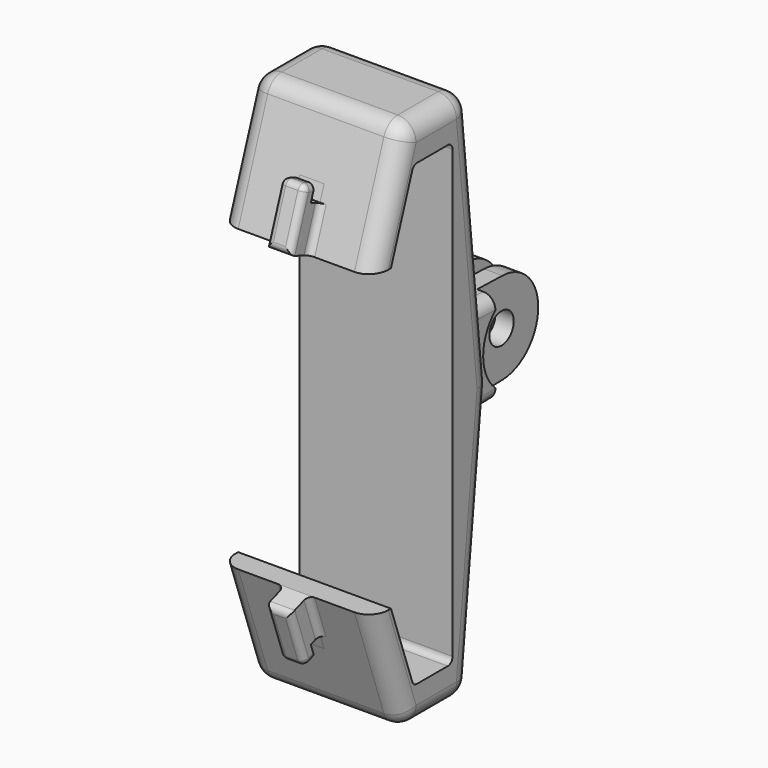
from build123d import *

# Parameters (mm, degrees)
F1_DEPTH      = 12.5
F3_DEPTH      = 7.5
F2_R          = 2.5
F4_DEPTH      = 4.5
F5_DEPTH      = 1.5
F6_R          = 3
F7_R          = 1.99999
F8_W          = 4
F8_H          = 7
F8_H_2        = 2.5
F9_DEPTH      = 4
F10_DEPTH     = 2
F11_T1_DEPTH  = 7
F11_T3_DEPTH  = 7
F11_T5_DEPTH  = 25
F11_T7_DEPTH  = 7
F11_T9_DEPTH  = 7
F11_T11_DEPTH = 9
F11_T13_DEPTH = 11
F11_T15_DEPTH = 2
F11_T17_DEPTH = 11
F11_T19_DEPTH = 11
F11_T21_DEPTH = 11
F11_T26_DEPTH = 1.02
F11_S31_W     = 1.02
F11_S31_H     = 1.02
F11_T32_DEPTH = 1.02
F11_T38_DEPTH = 1.02
F11_S43_W     = 1.02
F11_S43_H     = 1.02
F11_T44_DEPTH = 1.02
F11_T50_DEPTH = 3.5
F11_T55_DEPTH = 3.5
F11_T60_DEPTH = 3.5
F11_T65_DEPTH = 3.5


# Not quite as in the source:
# - a fillet or chamfer that OpenCascade refuses, or shapes differently, is made with other operations: its cross-section is extruded or revolved along the edge and cut away or added
# - two fillets or chamfers of one size are made in one step
# - a fillet or chamfer is up to 0.001 mm smaller than in the source, because OpenCascade refuses the exact size
# - a pattern or mirror of a feature is missing from the dataset's text; its kind, count and spacing are read off the source's solid


with BuildPart() as f1:
    # F0 (on Right) → F1 (new body, symmetric)
    with BuildSketch(Plane.YZ):
        Polygon((-8, 37.5), (0, 37.5), (0, -37.5), (-8, -37.5), (-12.6, -24.5), (-16.312652284, -24.5), (-9.589575361, -43.5), (3.5, -43.5), (8, 0), (3.5, 43.5), (-9.589575361, 43.5), (-16.312652284, 24.5), (-12.6, 24.5), align=None)
    extrude(amount=F1_DEPTH, both=True)

    # F2 (on Right) → F3 (join, symmetric)
    with BuildSketch(Plane.YZ):
        with BuildLine():
            ThreePointArc((15, -5.5901699437), (12.5, 0), (15, 5.5901699437))
            Line((15, 5.5901699437), (15, 7.6335005515))
            Line((15, 7.6335005515), (7.189168859, 7.8380343632))
            Line((7.189168859, 7.8380343632), (8, 0))
            Line((8, 0), (7.189168859, -7.8380343632))
            Line((7.189168859, -7.8380343632), (15, -7.6335005515))
            Line((15, -7.6335005515), (15, -5.5901699437))
        make_face()
    extrude(amount=F3_DEPTH, both=True)

    # F2 (on Right) → F4 (join, symmetric)
    with BuildSketch(Plane.YZ):
        with BuildLine():
            ThreePointArc((15, 5.5901699437), (17.4157731381, 7.0407223725), (20.1963271123, 7.4974299373))
            Line((20.1963271123, 7.4974299373), (15, 7.6335005515))
            Line((15, 7.6335005515), (15, 5.5901699437))
        make_face()
        with BuildLine():
            ThreePointArc((20.1963271123, -7.4974299373), (25.3722645757, -5.2334284488), (27.5, 0))
            ThreePointArc((27.5, 0), (25.3722645757, 5.2334284488), (20.1963271123, 7.4974299373))
            ThreePointArc((20.1963271123, 7.4974299373), (17.4157731381, 7.0407223725), (15, 5.5901699437))
            Line((15, 5.5901699437), (15, -5.5901699437))
            ThreePointArc((15, -5.5901699437), (17.4157731381, -7.0407223725), (20.1963271123, -7.4974299373))
        make_face()
        with Locations((20, 0)):
            Circle(F2_R, mode=Mode.SUBTRACT)
        with BuildLine():
            Line((15, -5.5901699437), (15, 5.5901699437))
            ThreePointArc((15, 5.5901699437), (12.5, 0), (15, -5.5901699437))
        make_face()
        with BuildLine():
            Line((15, -7.6335005515), (20.1963271123, -7.4974299373))
            ThreePointArc((20.1963271123, -7.4974299373), (17.4157731381, -7.0407223725), (15, -5.5901699437))
            Line((15, -5.5901699437), (15, -7.6335005515))
        make_face()
    extrude(amount=F4_DEPTH, both=True)

    # F2 (on Right) → F5 (cut, symmetric)
    with BuildSketch(Plane.YZ):
        with BuildLine():
            ThreePointArc((15, 5.5901699437), (17.4157731381, 7.0407223725), (20.1963271123, 7.4974299373))
            Line((20.1963271123, 7.4974299373), (15, 7.6335005515))
            Line((15, 7.6335005515), (15, 5.5901699437))
        make_face()
        with BuildLine():
            Line((15, -7.6335005515), (20.1963271123, -7.4974299373))
            ThreePointArc((20.1963271123, -7.4974299373), (17.4157731381, -7.0407223725), (15, -5.5901699437))
            Line((15, -5.5901699437), (15, -7.6335005515))
        make_face()
        with BuildLine():
            ThreePointArc((20.1963271123, -7.4974299373), (25.3722645757, -5.2334284488), (27.5, 0))
            ThreePointArc((27.5, 0), (25.3722645757, 5.2334284488), (20.1963271123, 7.4974299373))
            ThreePointArc((20.1963271123, 7.4974299373), (17.4157731381, 7.0407223725), (15, 5.5901699437))
            Line((15, 5.5901699437), (15, -5.5901699437))
            ThreePointArc((15, -5.5901699437), (17.4157731381, -7.0407223725), (20.1963271123, -7.4974299373))
        make_face()
        with Locations((20, 0)):
            Circle(F2_R, mode=Mode.SUBTRACT)
        with BuildLine():
            Line((15, -5.5901699437), (15, 5.5901699437))
            ThreePointArc((15, 5.5901699437), (12.5, 0), (15, -5.5901699437))
        make_face()
    extrude(amount=F5_DEPTH, both=True, mode=Mode.SUBTRACT)

    # F6
    f6_edges = [f1.edges().sort_by_distance(p)[0] for p in [
        (12.5, 5.75, 21.75),
        (12.5, 5.75, -21.75),
        (12.5, -3.044788, -43.5),
        (12.5, -12.951114, -34),
        (0, -9.589575, -43.5),
        (-12.5, -12.951114, -34),
        (-12.5, 5.75, -21.75),
        (-12.5, -3.044788, -43.5),
        (-12.5, 5.75, 21.75),
        (0, 3.5, 43.5),
        (0, 3.5, -43.5),
        (0, -9.589575, 43.5),
        (-12.5, -3.044788, 43.5),
        (-12.5, -12.951114, 34),
        (12.5, -12.951114, 34),
        (12.5, -3.044788, 43.5),
    ]]
    fillet(f6_edges, radius=F6_R)

    # F7 (radius 2 in the source; OpenCascade refuses exactly that, so slightly less here)
    f7_edges = [f1.edges().sort_by_distance(p)[0] for p in [
        (0, 7.189169, 7.838034),
        (-7.5, 7.594584, 3.919017),
        (-7.5, 7.594584, -3.919017),
        (0, 7.189169, -7.838034),
        (7.5, 7.594584, -3.919017),
        (7.5, 7.594584, 3.919017),
        (7.5, 11.094584, 7.735767),
        (7.5, 11.094584, -7.735767),
        (-7.5, 11.094584, -7.735767),
        (-7.5, 11.094584, 7.735767),
    ]]
    fillet(f7_edges, radius=F7_R)

    # F8 (on face) → F9 (join)
    with BuildSketch(Plane(origin=(0, -22.2020311107, -7.8561033161), x_dir=(1, 0, 0), z_dir=(0, -0.942722273, -0.3335786504))):
        with Locations((0, -21.155143154)):
            Rectangle(F8_W, F8_H)
        with Locations((0, -25.905143154)):
            Rectangle(F8_W, F8_H_2)
    f9 = extrude(amount=F9_DEPTH)

    # F9_copies: F9 across plane
    add(f9.mirror(Plane.XY))

    # F8 (on face) → F10 (cut)
    with BuildSketch(Plane(origin=(0, -22.2020311107, -7.8561033161), x_dir=(1, 0, 0), z_dir=(0, -0.942722273, -0.3335786504))):
        with Locations((0, -25.905143154)):
            Rectangle(F8_W, F8_H_2)
    f10 = extrude(amount=F10_DEPTH, mode=Mode.SUBTRACT)

    # F10_copies: F10 across plane
    add(f10.mirror(Plane.XY), mode=Mode.SUBTRACT)

    # F11: fillet of radius 1 on 20 edges, made by hand

    # F11_s2 → F11_t1 (join)
    with BuildSketch(Plane(origin=(0, 5.8893788266, -16.6438966839), x_dir=(1, 0, 0), z_dir=(0, 0.3335786504, -0.942722273))):
        with BuildLine():
            ThreePointArc((-3, 23.5509775753), (-2.2928932188, 23.8438707941), (-2, 24.5509775753))
            Line((-2, 24.5509775753), (-2, 23.5509775753))
            Line((-2, 23.5509775753), (-3, 23.5509775753))
        make_face()
    extrude(amount=F11_T1_DEPTH)

    # F11_s4 → F11_t3 (join)
    with BuildSketch(Plane(origin=(0, 8.2244293797, -23.2429525948), x_dir=(1, 0, 0), z_dir=(0, -0.3335786504, 0.942722273))):
        with BuildLine():
            ThreePointArc((3, -23.5509775753), (2.2928932188, -23.8438707941), (2, -24.5509775753))
            Line((2, -24.5509775753), (2, -23.5509775753))
            Line((2, -23.5509775753), (3, -23.5509775753))
        make_face()
    extrude(amount=F11_T3_DEPTH)

    # F11_s6 → F11_t5 (join)
    with BuildSketch(Plane.YZ.offset(-12.5)):
        with BuildLine():
            ThreePointArc((-8.2358106314, 36.8335786504), (-7.8703323924, 37.3165716902), (-7.2930883584, 37.5))
            Line((-7.2930883584, 37.5), (-8, 37.5))
            Line((-8, 37.5), (-8.2358106314, 36.8335786504))
        make_face()
        with BuildLine():
            ThreePointArc((-1, 37.5), (-0.2928932188, 37.2071067812), (0, 36.5))
            Line((0, 36.5), (0, 37.5))
            Line((0, 37.5), (-1, 37.5))
        make_face()
        with BuildLine():
            ThreePointArc((0, -36.5), (-0.2928932188, -37.2071067812), (-1, -37.5))
            Line((-1, -37.5), (0, -37.5))
            Line((0, -37.5), (0, -36.5))
        make_face()
        with BuildLine():
            ThreePointArc((-7.2930883584, -37.5), (-7.8703323924, -37.3165716902), (-8.2358106314, -36.8335786504))
            Line((-8.2358106314, -36.8335786504), (-8, -37.5))
            Line((-8, -37.5), (-7.2930883584, -37.5))
        make_face()
    extrude(amount=F11_T5_DEPTH)

    # F11_s8 → F11_t7 (join)
    with BuildSketch(Plane(origin=(0, 5.8893788266, 16.6438966839), x_dir=(1, 0, 0), z_dir=(0, 0.3335786504, 0.942722273))):
        with BuildLine():
            ThreePointArc((-3, -23.5509775753), (-2.2928932188, -23.8438707941), (-2, -24.5509775753))
            Line((-2, -24.5509775753), (-2, -23.5509775753))
            Line((-2, -23.5509775753), (-3, -23.5509775753))
        make_face()
    extrude(amount=F11_T7_DEPTH)

    # F11_s10 → F11_t9 (join)
    with BuildSketch(Plane(origin=(0, 8.2244293797, 23.2429525948), x_dir=(1, 0, 0), z_dir=(0, -0.3335786504, -0.942722273))):
        with BuildLine():
            ThreePointArc((3, 23.5509775753), (2.2928932188, 23.8438707941), (2, 24.5509775753))
            Line((2, 24.5509775753), (2, 23.5509775753))
            Line((2, 23.5509775753), (3, 23.5509775753))
        make_face()
    extrude(amount=F11_T9_DEPTH)

    # F11_s12 → F11_t11 (cut)
    with BuildSketch(Plane.YZ.offset(-4.5)):
        with BuildLine():
            ThreePointArc((-19.140819103, -25.5007359513), (-19.7097214903, -26.0127286381), (-19.7499627255, -26.7770368747))
            Line((-19.7499627255, -26.7770368747), (-20.083541376, -25.8343146018))
            Line((-20.083541376, -25.8343146018), (-19.140819103, -25.5007359513))
        make_face()
        with BuildLine():
            ThreePointArc((-19.140819103, 25.5007359513), (-19.7097214903, 26.0127286381), (-19.7499627255, 26.7770368747))
            Line((-19.7499627255, 26.7770368747), (-20.083541376, 25.8343146018))
            Line((-20.083541376, 25.8343146018), (-19.140819103, 25.5007359513))
        make_face()
    extrude(amount=F11_T11_DEPTH, mode=Mode.SUBTRACT)

    # F11_s14 → F11_t13 (cut)
    with BuildSketch(Plane(origin=(0, 5.0554322005, -14.2870910015), x_dir=(1, 0, 0), z_dir=(0, 0.3335786504, -0.942722273))):
        with BuildLine():
            ThreePointArc((-2, 26.5509775753), (-1.7071067812, 27.2580843565), (-1, 27.5509775753))
            Line((-1, 27.5509775753), (-2, 27.5509775753))
            Line((-2, 27.5509775753), (-2, 26.5509775753))
        make_face()
    extrude(amount=F11_T13_DEPTH, mode=Mode.SUBTRACT)

    # F11_s16 → F11_t15 (cut)
    with BuildSketch(Plane.YZ.offset(-1)):
        with BuildLine():
            ThreePointArc((-15.9718219238, -34.4565975446), (-16.7361301605, -34.4163563094), (-17.2481228472, -33.8474539221))
            Line((-17.2481228472, -33.8474539221), (-16.9145441968, -34.7901761951))
            Line((-16.9145441968, -34.7901761951), (-15.9718219238, -34.4565975446))
        make_face()
        with BuildLine():
            ThreePointArc((-15.9718219238, 34.4565975446), (-16.7361301605, 34.4163563094), (-17.2481228472, 33.8474539221))
            Line((-17.2481228472, 33.8474539221), (-16.9145441968, 34.7901761951))
            Line((-16.9145441968, 34.7901761951), (-15.9718219238, 34.4565975446))
        make_face()
    extrude(amount=F11_T15_DEPTH, mode=Mode.SUBTRACT)

    # F11_s18 → F11_t17 (cut)
    with BuildSketch(Plane(origin=(0, 8.7247973553, -24.6570360042), x_dir=(1, 0, 0), z_dir=(0, -0.3335786504, 0.942722273))):
        with BuildLine():
            ThreePointArc((1, -27.5509775753), (1.7071067812, -27.2580843565), (2, -26.5509775753))
            Line((2, -26.5509775753), (2, -27.5509775753))
            Line((2, -27.5509775753), (1, -27.5509775753))
        make_face()
    extrude(amount=F11_T17_DEPTH, mode=Mode.SUBTRACT)

    # F11_s20 → F11_t19 (cut)
    with BuildSketch(Plane(origin=(0, 8.7247973553, 24.6570360042), x_dir=(1, 0, 0), z_dir=(0, -0.3335786504, -0.942722273))):
        with BuildLine():
            ThreePointArc((1, 27.5509775753), (1.7071067812, 27.2580843565), (2, 26.5509775753))
            Line((2, 26.5509775753), (2, 27.5509775753))
            Line((2, 27.5509775753), (1, 27.5509775753))
        make_face()
    extrude(amount=F11_T19_DEPTH, mode=Mode.SUBTRACT)

    # F11_s22 → F11_t21 (cut)
    with BuildSketch(Plane(origin=(0, 5.0554322005, 14.2870910015), x_dir=(1, 0, 0), z_dir=(0, 0.3335786504, 0.942722273))):
        with BuildLine():
            ThreePointArc((-2, -26.5509775753), (-1.7071067812, -27.2580843565), (-1, -27.5509775753))
            Line((-1, -27.5509775753), (-2, -27.5509775753))
            Line((-2, -27.5509775753), (-2, -26.5509775753))
        make_face()
    extrude(amount=F11_T21_DEPTH, mode=Mode.SUBTRACT)


with BuildPart() as f11_tool24:
    # F11_s25 → F11_t26 (new body)
    with BuildSketch(Plane.YZ.offset(-1)):
        Polygon((-16.3054005743, -33.5138752716), (-15.9651503508, -34.4754519901), (-16.9267270692, -34.8157022135), (-17.2669772927, -33.8541254951), align=None)
    extrude(amount=-F11_T26_DEPTH)

    # F11_s27 → F11_t28 (revolve, cut)
    with BuildSketch(Plane(origin=(-1, -16.3054005743, -33.5138752716), x_dir=(0, 0.4307295862, 0.9024810378), z_dir=(0, -0.9024810378, 0.4307295862))):
        with BuildLine():
            ThreePointArc((0, -1), (1, 0), (0, 1))
            Line((0, 1), (0, -1))
        make_face()
    revolve(axis=Axis((-1, -16.3054005743, -33.5138752716), (-1, 0, 0)), mode=Mode.SUBTRACT)


with BuildPart() as f1_1:
    add(f1.part)

    # F11_t23: cut F11_tool24
    add(f11_tool24.part, mode=Mode.SUBTRACT)


with BuildPart() as f11_tool30:
    # F11_s31 → F11_t32 (new body)
    with BuildSketch(Plane(origin=(0, 8.7247973553, -24.6570360042), x_dir=(1, 0, 0), z_dir=(0, 0.3335786504, -0.942722273))):
        with Locations((1.51, 27.0609775753)):
            Rectangle(F11_S31_W, F11_S31_H)
    extrude(amount=F11_T32_DEPTH)

    # F11_s33 → F11_t34 (revolve, cut)
    with BuildSketch(Plane(origin=(1, -16.3054005743, -33.5138752716), x_dir=(-0.7071067812, 0.666605312, 0.2358757258), z_dir=(-0.7071067812, -0.666605312, -0.2358757258))):
        with BuildLine():
            ThreePointArc((0, -1), (1, 0), (0, 1))
            Line((0, 1), (0, -1))
        make_face()
    revolve(axis=Axis((1, -16.3054005743, -33.5138752716), (0, 0.3335786504, -0.942722273)), mode=Mode.SUBTRACT)


with BuildPart() as f1_2:
    add(f1_1.part)

    # F11_t29: cut F11_tool30
    add(f11_tool30.part, mode=Mode.SUBTRACT)


with BuildPart() as f11_tool36:
    # F11_s37 → F11_t38 (new body)
    with BuildSketch(Plane.YZ.offset(1)):
        Polygon((-16.3054005743, 33.5138752716), (-15.9651503508, 34.4754519901), (-16.9267270692, 34.8157022135), (-17.2669772927, 33.8541254951), align=None)
    extrude(amount=F11_T38_DEPTH)

    # F11_s39 → F11_t40 (revolve, cut)
    with BuildSketch(Plane(origin=(1, -16.3054005743, 33.5138752716), x_dir=(0, 0.4307295862, -0.9024810378), z_dir=(0, -0.9024810378, -0.4307295862))):
        with BuildLine():
            ThreePointArc((0, -1), (1, 0), (0, 1))
            Line((0, 1), (0, -1))
        make_face()
    revolve(axis=Axis((1, -16.3054005743, 33.5138752716), (1, 0, 0)), mode=Mode.SUBTRACT)


with BuildPart() as f1_3:
    add(f1_2.part)

    # F11_t35: cut F11_tool36
    add(f11_tool36.part, mode=Mode.SUBTRACT)


with BuildPart() as f11_tool42:
    # F11_s43 → F11_t44 (new body)
    with BuildSketch(Plane(origin=(0, 8.7247973553, 24.6570360042), x_dir=(1, 0, 0), z_dir=(0, 0.3335786504, 0.942722273))):
        with Locations((-1.51, -27.0609775753)):
            Rectangle(F11_S43_W, F11_S43_H)
    extrude(amount=F11_T44_DEPTH)

    # F11_s45 → F11_t46 (revolve, cut)
    with BuildSketch(Plane(origin=(-1, -16.3054005743, 33.5138752716), x_dir=(0.7071067812, 0.666605312, -0.2358757258), z_dir=(0.7071067812, -0.666605312, 0.2358757258))):
        with BuildLine():
            ThreePointArc((0, -1), (1, 0), (0, 1))
            Line((0, 1), (0, -1))
        make_face()
    revolve(axis=Axis((-1, -16.3054005743, 33.5138752716), (0, 0.3335786504, 0.942722273)), mode=Mode.SUBTRACT)


with BuildPart() as f1_4:
    add(f1_3.part)

    # F11_t41: cut F11_tool42
    add(f11_tool42.part, mode=Mode.SUBTRACT)


with BuildPart() as f11_tool48:
    # F11_s49 → F11_t50 (new body)
    with BuildSketch(Plane(origin=(0, -21.7306699742, -7.6893139909), x_dir=(1, 0, 0), z_dir=(0, -0.942722273, -0.3335786504))):
        with BuildLine():
            ThreePointArc((1, -27.155143154), (1.7071067812, -26.8622499352), (2, -26.155143154))
            Line((2, -26.155143154), (2, -27.155143154))
            Line((2, -27.155143154), (1, -27.155143154))
        make_face()
    extrude(amount=F11_T50_DEPTH)

    split(bisect_by=Plane(origin=(0, -22.2020311107, -7.8561033161), x_dir=(1, 0, 0), z_dir=(0, -0.942722273, -0.3335786504)), keep=Keep.TOP)


with BuildPart() as f1_5:
    add(f1_4.part)

    # F11_t47: cut F11_tool48
    add(f11_tool48.part, mode=Mode.SUBTRACT)


with BuildPart() as f11_tool53:
    # F11_s54 → F11_t55 (new body)
    with BuildSketch(Plane(origin=(0, -21.7306699742, -7.6893139909), x_dir=(1, 0, 0), z_dir=(0, -0.942722273, -0.3335786504))):
        with BuildLine():
            ThreePointArc((-2, -26.155143154), (-1.7071067812, -26.8622499352), (-1, -27.155143154))
            Line((-1, -27.155143154), (-2, -27.155143154))
            Line((-2, -27.155143154), (-2, -26.155143154))
        make_face()
    extrude(amount=F11_T55_DEPTH)

    split(bisect_by=Plane(origin=(0, -22.2020311107, -7.8561033161), x_dir=(1, 0, 0), z_dir=(0, -0.942722273, -0.3335786504)), keep=Keep.TOP)


with BuildPart() as f1_6:
    add(f1_5.part)

    # F11_t52: cut F11_tool53
    add(f11_tool53.part, mode=Mode.SUBTRACT)


with BuildPart() as f11_tool58:
    # F11_s59 → F11_t60 (new body)
    with BuildSketch(Plane(origin=(0, -21.7306699742, 7.6893139909), x_dir=(1, 0, 0), z_dir=(0, -0.942722273, 0.3335786504))):
        with BuildLine():
            ThreePointArc((1, 27.155143154), (1.7071067812, 26.8622499352), (2, 26.155143154))
            Line((2, 26.155143154), (2, 27.155143154))
            Line((2, 27.155143154), (1, 27.155143154))
        make_face()
    extrude(amount=F11_T60_DEPTH)

    split(bisect_by=Plane(origin=(0, -22.2020311107, 7.8561033161), x_dir=(1, 0, 0), z_dir=(0, -0.942722273, 0.3335786504)), keep=Keep.TOP)


with BuildPart() as f1_7:
    add(f1_6.part)

    # F11_t57: cut F11_tool58
    add(f11_tool58.part, mode=Mode.SUBTRACT)


with BuildPart() as f11_tool63:
    # F11_s64 → F11_t65 (new body)
    with BuildSketch(Plane(origin=(0, -21.7306699742, 7.6893139909), x_dir=(1, 0, 0), z_dir=(0, -0.942722273, 0.3335786504))):
        with BuildLine():
            ThreePointArc((-1, 27.155143154), (-1.7071067812, 26.8622499352), (-2, 26.155143154))
            Line((-2, 26.155143154), (-2, 27.155143154))
            Line((-2, 27.155143154), (-1, 27.155143154))
        make_face()
    extrude(amount=F11_T65_DEPTH)

    split(bisect_by=Plane(origin=(0, -22.2020311107, 7.8561033161), x_dir=(1, 0, 0), z_dir=(0, -0.942722273, 0.3335786504)), keep=Keep.TOP)


with BuildPart() as f1_8:
    add(f1_7.part)

    # F11_t62: cut F11_tool63
    add(f11_tool63.part, mode=Mode.SUBTRACT)


solid = f1_8.part
